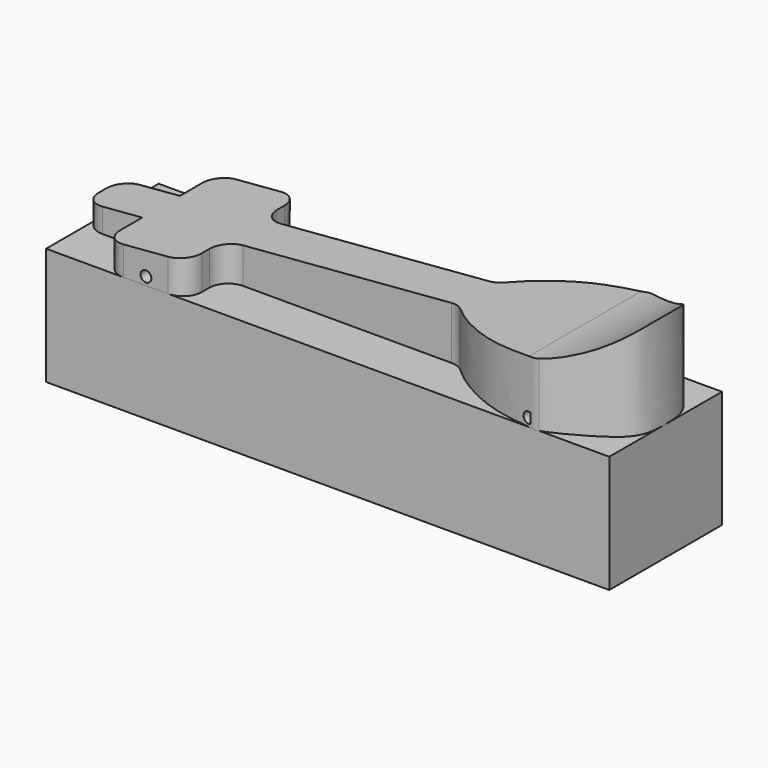
from build123d import *

# Parameters (mm, degrees)
F0_W      = 152.4
F0_H      = 38.1
F1_DEPTH  = 31.75
F3_DEPTH  = 28.575
F4_R      = 5.08
F7_DEPTH  = 80.518
F10_R     = 1.4605
F12_DEPTH = 38.2592987687
F11_R     = 1.4605
F13_DEPTH = 38.2592987687


# Not quite as in the source:
# - two fillets or chamfers of one size are made in one step


with BuildPart() as f1:
    # F0 (on Top) → F1 (new body)
    with BuildSketch(Plane.XY):
        Rectangle(F0_W, F0_H)
    extrude(amount=F1_DEPTH)


with BuildPart() as f3:
    # F2 (on face) → F3 (new body)
    with BuildSketch(Plane.XY.offset(31.75)):
        with BuildLine():
            Line((-76.2, 0), (-76.2, -6.35))
            Line((-76.2, -6.35), (-60.325, -6.35))
            Line((-60.325, -6.35), (-60.325, -19.05))
            Line((-60.325, -19.05), (-38.1, -19.05))
            Line((-38.1, -19.05), (-38.1, -6.35))
            Line((-38.1, -6.35), (25.4, -6.35))
            add(Edge.make_bspline(
                [(25.4, -6.35), (30.1994255175, -11.3051086915), (42.1205172368, -18.1239943856), (54.9564309447, -18.8622083385), (56.1841019589, -19.3262532215), (57.17600137, -19.05)],
                knots=[0, 0, 0, 0, 0.2462330157, 0.4286545069, 0.5090961206, 0.5090961206, 0.5090961206, 0.5090961206], degree=3))
            add(Edge.make_bspline(
                [(57.17600137, -19.05), (59.7234135096, -18.3405220002), (71.0893380416, -12.3784866134), (75.9140076642, -6.9880877245), (76.2, -2.0431288688), (76.2, 0)],
                knots=[0.5090961206, 0.5090961206, 0.5090961206, 0.5090961206, 0.7156875762, 0.8642372546, 1, 1, 1, 1], degree=3))
            add(Edge.make_bspline(
                [(25.4, 6.35), (30.1994255175, 11.3051086915), (42.1205172368, 18.1239943856), (54.9564309447, 18.8622083385), (57.1489628968, 19.6909590555), (71.0893380416, 12.3784866134), (75.9140076642, 6.9880877245), (76.2, 2.0431288688), (76.2, 0)],
                knots=[0, 0, 0, 0, 0.2462330157, 0.4286545069, 0.5090961206, 0.7156875762, 0.8642372546, 1, 1, 1, 1], degree=3))
            Line((25.4, 6.35), (-38.1, 6.35))
            Line((-38.1, 6.35), (-38.1, 19.05))
            Line((-38.1, 19.05), (-60.325, 19.05))
            Line((-60.325, 19.05), (-60.325, 6.35))
            Line((-60.325, 6.35), (-76.2, 6.35))
            Line((-76.2, 6.35), (-76.2, 0))
        make_face()
    extrude(amount=F3_DEPTH)

    # F4
    f4_edges = [f3.edges().sort_by_distance(p)[0] for p in [
        (-76.2, -6.35, 46.0375),
        (-60.325, -19.05, 46.0375),
        (-38.1, -19.05, 46.0375),
        (-38.1, -6.35, 46.0375),
        (-76.2, 6.35, 46.0375),
        (-60.325, 19.05, 46.0375),
        (-38.1, 19.05, 46.0375),
        (-38.1, 6.35, 46.0375),
        (25.4, 6.35, 46.0375),
        (25.4, -6.35, 46.0375),
    ]]
    fillet(f4_edges, radius=F4_R)

    # F6 (on Front) → F7 (cut, symmetric)
    with BuildSketch(Plane.XZ):
        with BuildLine():
            Line((-86.506019904, 62.4197835069), (-86.506019904, 37.0197835069))
            Line((-86.506019904, 37.0197835069), (54.4187102132, 48.6035190311))
            ThreePointArc((54.4187102132, 48.6035190311), (67.7020293118, 52.1879415791), (78.8461435109, 60.2566075157))
            Line((78.8461435109, 60.2566075157), (79.1688337922, 60.5943761766))
            Line((79.1688337922, 60.5943761766), (-86.506019904, 62.4197835069))
        make_face()
    extrude(amount=F7_DEPTH, both=True, mode=Mode.SUBTRACT)

    # F10 (on face) → F12 (cut, through all)
    with BuildSketch(Plane.XZ.offset(19.05)):
        with Locations((-49.1822399199, 33.9363620336)):
            Circle(F10_R)
    extrude(amount=-F12_DEPTH, mode=Mode.SUBTRACT)

    # F11 (on face) → F13 (cut, through all)
    with BuildSketch(Plane.XZ.offset(19.05)):
        with Locations((54.2619526386, 33.9150123949)):
            Circle(F11_R)
    extrude(amount=-F13_DEPTH, mode=Mode.SUBTRACT)


solid = Compound([f1.part, f3.part])
